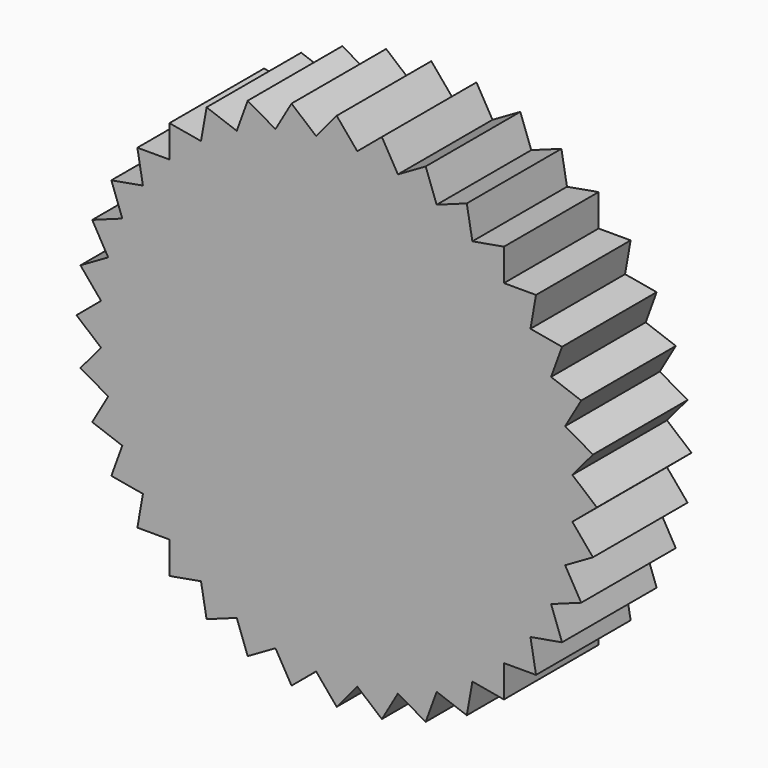
from build123d import *

# Parameters (mm, degrees)
F0_R            = 50.8
F1_DEPTH        = 25.4
F3_DEPTH        = 25.4
F3_COPIES_COUNT = 36


# Not quite as in the source:
# - a pattern or mirror of a feature is missing from the dataset's text; its kind, count and spacing are read off the source's solid


with BuildPart() as f1:
    # F0 (on Front) → F1 (new body)
    with BuildSketch(Plane.XZ):
        Circle(F0_R)
    extrude(amount=F1_DEPTH)

    # F2 (on Front) → F3 (join, through all)
    with BuildSketch(Plane.XZ):
        Polygon((4.4275117316, 50.6066906631), (0, 55.88), (-4.4275117316, 50.6066906631), align=None)
    f3 = extrude(amount=F3_DEPTH)

    # F3_copies: F3 ×36 about axis
    f3_copies_axis = Axis((0, 0, 0), (0, 1, 0))
    for i in range(1, F3_COPIES_COUNT):
        add(f3.rotate(f3_copies_axis, i * 360 / F3_COPIES_COUNT))


solid = f1.part
